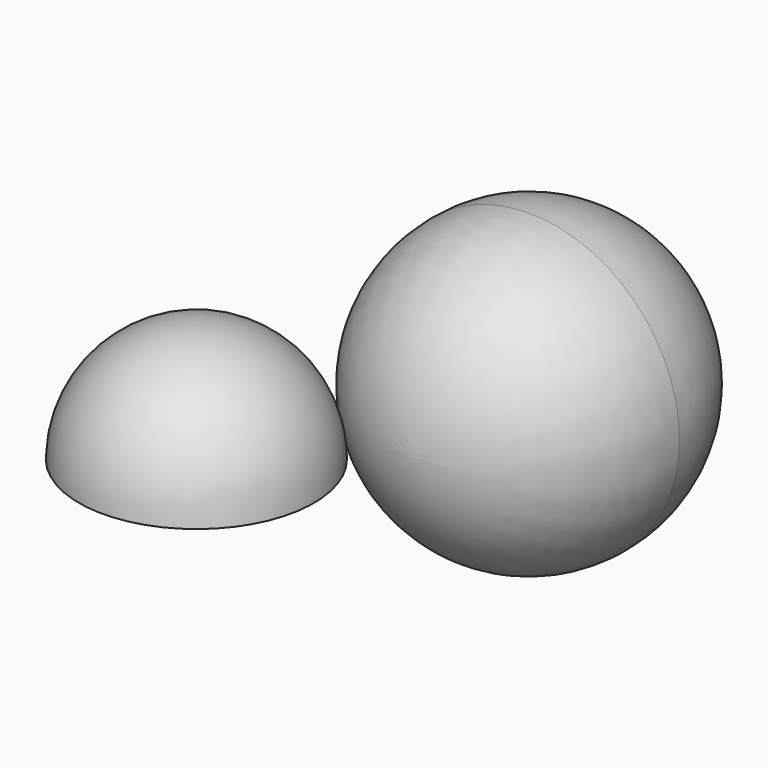
from build123d import *

# Parameters (mm, degrees)
F3_ANGLE = 182.8582129334


with BuildPart() as f1:
    # F0 (on Top) → F1 (revolve)
    with BuildSketch(Plane.XY):
        with BuildLine():
            ThreePointArc((-26.1427345622, -10.0239053509), (-0.760386555, 0.6157664986), (9.7360185112, 26.0576942578))
            ThreePointArc((9.7360185112, 26.0576942578), (-0.760386555, 51.4996220171), (-26.1427345622, 62.1392938666))
            Line((-26.1427345622, 62.1392938666), (-26.1427345622, -10.0239053509))
        make_face()
    revolve(axis=Axis((-26.1427345622, 26.0576942578, 0), (0, -1, 0)))


with BuildPart() as f3:
    # F2 (on Top) → F3 (revolve)
    with BuildSketch(Plane.XY):
        with BuildLine():
            Line((-38.6602226546, -14.0395503166), (-72.2698077066, -58.8833214605))
            ThreePointArc((-72.2698077066, -58.8833214605), (-33.0431296086, -53.2662284146), (-38.6602226546, -14.0395503166))
        make_face()
    revolve(axis=Axis((-55.4650151806, -36.4614358886, 0), (-0.5997345224, -0.8001990394, 0)), revolution_arc=F3_ANGLE)


solid = Compound([f1.part, f3.part])
